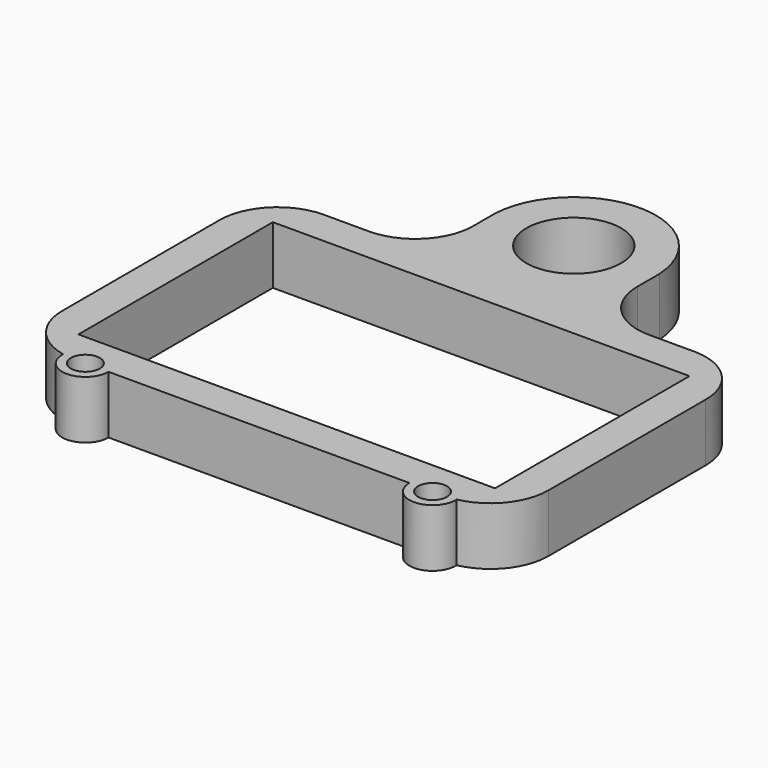
from build123d import *

# Parameters (mm, degrees)
F0_W     = 36
F0_H     = 21
F0_R     = 4.1
F1_DEPTH = 5
F2_R     = 5
F4_DEPTH = 5
F5_R     = 1.25
F6_DEPTH = 5


# Not quite as in the source:
# - a pattern or mirror of a feature is missing from the dataset's text; its kind, count and spacing are read off the source's solid


with BuildPart() as f1:
    # F0 (on Top) → F1 (new body)
    with BuildSketch(Plane.XY):
        with BuildLine():
            Line((-21, 13.5), (-21, 10.5))
            Line((-21, 10.5), (-21, -13.5))
            Line((-21, -13.5), (21, -13.5))
            Line((21, -13.5), (21, 10.5))
            Line((21, 10.5), (21.0088081658, 13.5))
            Line((21.0088081658, 13.5), (7.0901421979, 13.5))
            Line((7.0901421979, 13.5), (7.0901421979, 20.8740101776))
            ThreePointArc((7.0901421979, 20.8740101776), (0, 27.6), (-7.0901421979, 20.8740101776))
            Line((-7.0901421979, 20.8740101776), (-7.0901421979, 13.5))
            Line((-7.0901421979, 13.5), (-21, 13.5))
        make_face()
        Rectangle(F0_W, F0_H, mode=Mode.SUBTRACT)
        with Locations((0, 20.5)):
            Circle(F0_R, mode=Mode.SUBTRACT)
    extrude(amount=F1_DEPTH)

    # F2
    f2_edges = [f1.edges().sort_by_distance(p)[0] for p in [
        (-7.090142, 13.5, 2.5),
        (7.090142, 13.5, 2.5),
        (21.008808, 13.5, 2.5),
        (-21, 13.5, 2.5),
        (-21, -13.5, 2.5),
        (21, -13.5, 2.5),
    ]]
    fillet(f2_edges, radius=F2_R)

    # F3 (on face) → F4 (join, through all)
    with BuildSketch(Plane.XY.offset(5)):
        with BuildLine():
            ThreePointArc((-16.9974730705, -13.3994946141), (-15.0502685736, -15.4993681678), (-13, -13.5))
            Line((-13, -13.5), (-16, -13.5))
            ThreePointArc((-16, -13.5), (-16.5012618724, -13.4748102009), (-16.9974730705, -13.3994946141))
        make_face()
    f4 = extrude(amount=-F4_DEPTH)

    # F4_copies: F4 across plane
    add(f4.mirror(Plane(origin=(0, 0, 0), x_dir=(0, 0, 1), z_dir=(1, 0, 0))))

    # F5 (on face) → F6 (cut, through all)
    with BuildSketch(Plane.XY.offset(5)):
        with Locations((-15, -13.5)):
            Circle(F5_R)
    f6 = extrude(amount=-F6_DEPTH, mode=Mode.SUBTRACT)

    # F6_copies: F6 across plane
    add(f6.mirror(Plane(origin=(0, 0, 0), x_dir=(0, 0, 1), z_dir=(1, 0, 0))), mode=Mode.SUBTRACT)


solid = f1.part
